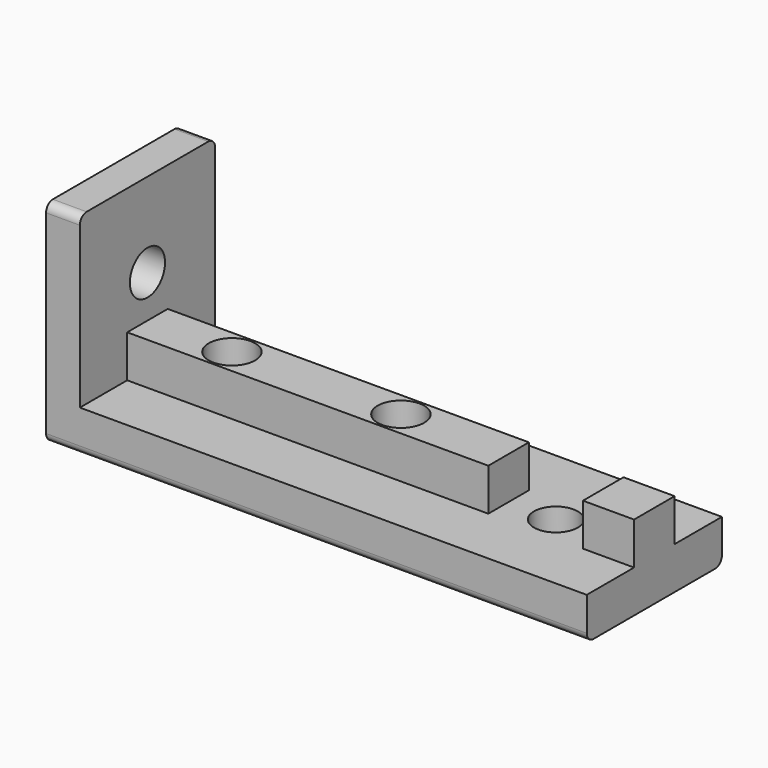
from build123d import *

# Parameters (mm, degrees)
F0_W         = 60
F0_H         = 20
F1_DEPTH     = 5
F2_W         = 60
F2_H         = 6
F3_DEPTH     = 5
F4_R         = 2.75
F5_DEPTH     = 25
F6_W         = 11.2
F6_H         = 6
F7_DEPTH     = 5
F8_R         = 2.6
F9_DEPTH     = 5
F10_R        = 2.6
F11_DEPTH    = 4
F12_R        = 1
F13_C1_SIZE2 = 0.5
F13_C1_SIZE  = 0.2886751346
F13_C2_SIZE2 = 0.5
F13_C2_SIZE  = 0.2886751346


# Not quite as in the source:
# - a feature names something its author has since deleted; it is built from what else it names


with BuildPart() as f1:
    # F0 (on Top) → F1 (new body)
    with BuildSketch(Plane.XY):
        with Locations((30, 0)):
            Rectangle(F0_W, F0_H)
    extrude(amount=F1_DEPTH)

    # F2 (on face) → F3 (join)
    with BuildSketch(Plane.XY.offset(5)):
        with Locations((30, 0)):
            Rectangle(F2_W, F2_H)
    extrude(amount=F3_DEPTH)

    # F4 (on face) → F5 (cut)
    with BuildSketch(Plane.XY.offset(10)):
        with Locations((30, 0)):
            Circle(F4_R)
        with Locations((10, 0)):
            Circle(F4_R)
    extrude(amount=-F5_DEPTH, mode=Mode.SUBTRACT)

    # F6 (on face) → F7 (cut, through all)
    with BuildSketch(Plane.XY.offset(10)):
        with Locations((48.35, 0)):
            Rectangle(F6_W, F6_H)
    extrude(amount=-F7_DEPTH, mode=Mode.SUBTRACT)

    # F8 (on face) → F9 (cut, through all)
    with BuildSketch(Plane.XY.offset(5)):
        with Locations((48.35, 0)):
            Circle(F8_R)
    extrude(amount=-F9_DEPTH, mode=Mode.SUBTRACT)

    # F10 (on face) → F11 (join)
    with BuildSketch(Plane(origin=(0, 0, 0), x_dir=(0, -1, 0), z_dir=(-1, 0, 0))):
        Polygon((-10, 25), (-10, 5), (-3, 5), (-3, 10), (3, 10), (3, 5), (10, 5), (10, 25), align=None)
        with Locations((0, 15)):
            Circle(F10_R, mode=Mode.SUBTRACT)
        Polygon((-10, 5), (-10, 0), (10, 0), (10, 5), (3, 5), (3, 10), (-3, 10), (-3, 5), align=None)
    extrude(amount=F11_DEPTH)

    # F12
    f12_edges = [f1.edges().sort_by_distance(p)[0] for p in [
        (-2, -10, 25),
        (-2, 10, 25),
        (28, -10, 0),
        (28, 10, 0),
    ]]
    fillet(f12_edges, radius=F12_R)

    # F13: chamfer of 0.5 x 0.2886751346 on 2 edges, made by hand

    # F13_c1
    f13_c1_edges = [f1.edges().sort_by_distance(p)[0] for p in [
        (7.25, 0, 0),
    ]]
    f13_c1_side = f1.faces().sort_by_distance((7.2442264973, 0, 0))[0]
    chamfer(f13_c1_edges, length=F13_C1_SIZE, length2=F13_C1_SIZE2, reference=f13_c1_side)

    # F13_c2
    f13_c2_edges = [f1.edges().sort_by_distance(p)[0] for p in [
        (27.25, 0, 0),
    ]]
    f13_c2_side = f1.faces().sort_by_distance((27.2442264973, 0, 0))[0]
    chamfer(f13_c2_edges, length=F13_C2_SIZE, length2=F13_C2_SIZE2, reference=f13_c2_side)


solid = f1.part
